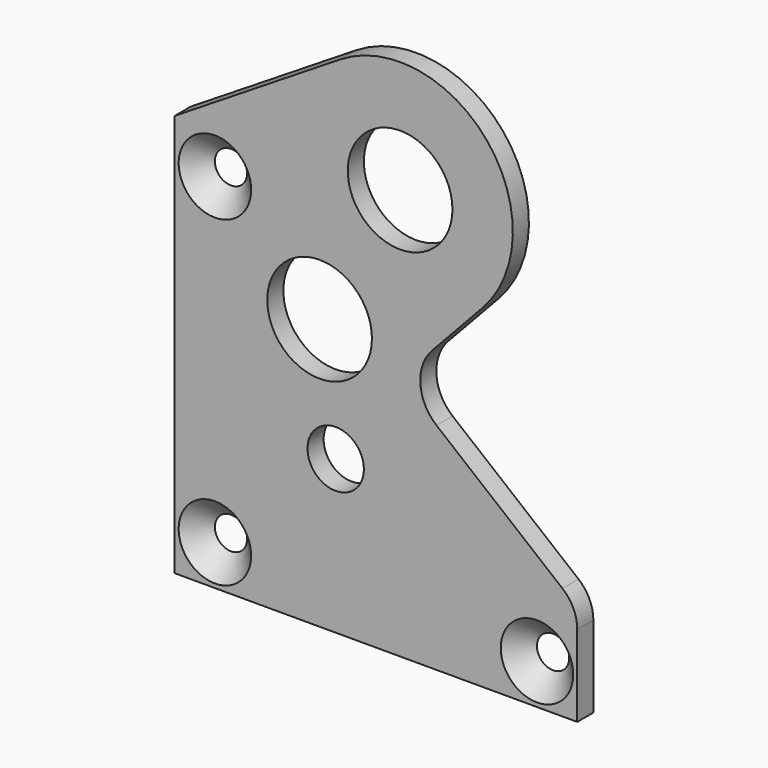
from build123d import *

# Parameters (mm, degrees)
F0_R     = 4
F0_R_2   = 7
F0_R_3   = 13
F1_DEPTH = 5
F2_SIZE  = 4.99999
F3_R     = 10


# Not quite as in the source:
# - a fillet or chamfer is up to 0.001 mm smaller than in the source, because OpenCascade refuses the exact size


with BuildPart() as f1:
    # F0 (on Front) → F1 (new body)
    with BuildSketch(Plane.XZ):
        with BuildLine():
            Line((0, 100), (0, 0))
            Line((0, 0), (100, 0))
            Line((100, 0), (100, 25))
            Line((100, 25), (65.0521931045, 53.4719299169))
            ThreePointArc((65.0521931045, 53.4719299169), (61.0252955601, 61.2544381602), (63.9626496251, 69.51005985))
            Line((63.9626496251, 69.51005985), (76.4587100452, 82.8834840181))
            ThreePointArc((76.4587100452, 82.8834840181), (77.6106511533, 119.803925318), (41.1521770426, 125.7390428077))
            Line((41.1521770426, 125.7390428077), (0, 100))
        make_face()
        with Locations((10, 10)):
            Circle(F0_R, mode=Mode.SUBTRACT)
        with Locations((40, 38)):
            Circle(F0_R_2, mode=Mode.SUBTRACT)
        with Locations((90, 10)):
            Circle(F0_R, mode=Mode.SUBTRACT)
        with Locations((10, 90)):
            Circle(F0_R, mode=Mode.SUBTRACT)
        with Locations((36, 67.24)):
            Circle(F0_R_3, mode=Mode.SUBTRACT)
        with Locations((56, 102)):
            Circle(F0_R_3, mode=Mode.SUBTRACT)
    extrude(amount=F1_DEPTH)

    # F2 (size 5 in the source; OpenCascade refuses exactly that, so slightly less here)
    f2_edges = [f1.edges().sort_by_distance(p)[0] for p in [
        (6, -5, 10),
        (86, -5, 10),
        (6, -5, 90),
    ]]
    chamfer(f2_edges, length=F2_SIZE)

    # F3
    f3_edges = [f1.edges().sort_by_distance(p)[0] for p in [
        (100, -2.5, 25),
    ]]
    fillet(f3_edges, radius=F3_R)


solid = f1.part
